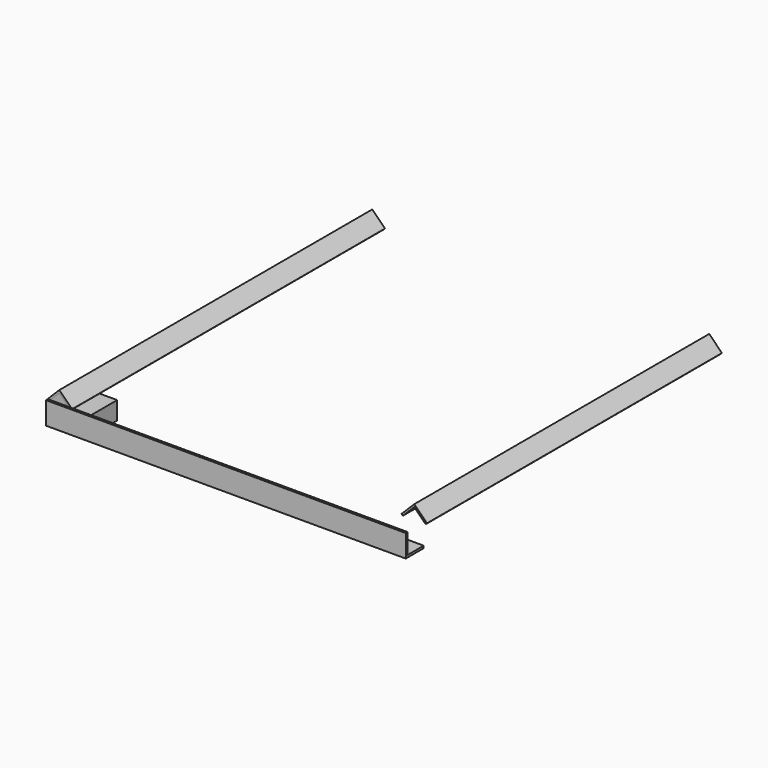
from build123d import *

# Parameters (mm, degrees)
F1_DEPTH = 205
F2_DEPTH = 25
F4_DEPTH = 40
F6_DEPTH = 400


# Not quite as in the source:
# - a pattern or mirror of a feature is missing from the dataset's text; its kind, count and spacing are read off the source's solid


with BuildPart() as f1:
    # F0 (on Front) → F1 (new body, symmetric)
    with BuildSketch(Plane.XZ):
        Polygon((-174.6419423149, -1.4142135624), (-173.2277287525, 0), (-187.3698643763, 14.1421356237), (-201.512, 0), (-200.0977864376, -1.4142135624), (-187.3698643763, 11.313708499), align=None)
    extrude(amount=F1_DEPTH, both=True)


with BuildPart() as f1_copies_1:
    # F1_copies: instance of F1
    add(f1.part.mirror(Plane(origin=(0, 0, 0), x_dir=(0, 0, 1), z_dir=(1, 0, 0))))


with BuildPart() as f1_1:
    add(f1.part)

    # F2 (add): a face of the model
    f2_faces = [f1_1.faces().sort_by_distance(p)[0] for p in [
        (-174.1630897779, -205, -0.478852537),
    ]]
    extrude(f2_faces, amount=F2_DEPTH)


with BuildPart() as f4:
    # F3 (on face) → F4 (new body)
    with BuildSketch(Plane.XZ.offset(230)):
        Polygon((-174.6419423149, -1.4142135624), (-187.3698643763, 11.313708499), (-200.0977864376, -1.4142135624), (-200.0977864376, -21.4142135624), (-155, -21.4142135624), (-155, -1.4142135624), align=None)
    extrude(amount=-F4_DEPTH)


with BuildPart() as f6:
    # F5 (on face) → F6 (new body)
    with BuildSketch(Plane(origin=(-200.0977864376, 0, 0), x_dir=(0, -1, 0), z_dir=(-1, 0, 0))):
        Polygon((230, 1.0857864376), (230, -21.4142135624), (207.5, -21.4142135624), (207.5, -23.9142135624), (232.5, -23.9142135624), (232.5, 1.0857864376), align=None)
    extrude(amount=-F6_DEPTH)


solid = Compound([f1_copies_1.part, f1_1.part, f4.part, f6.part])
